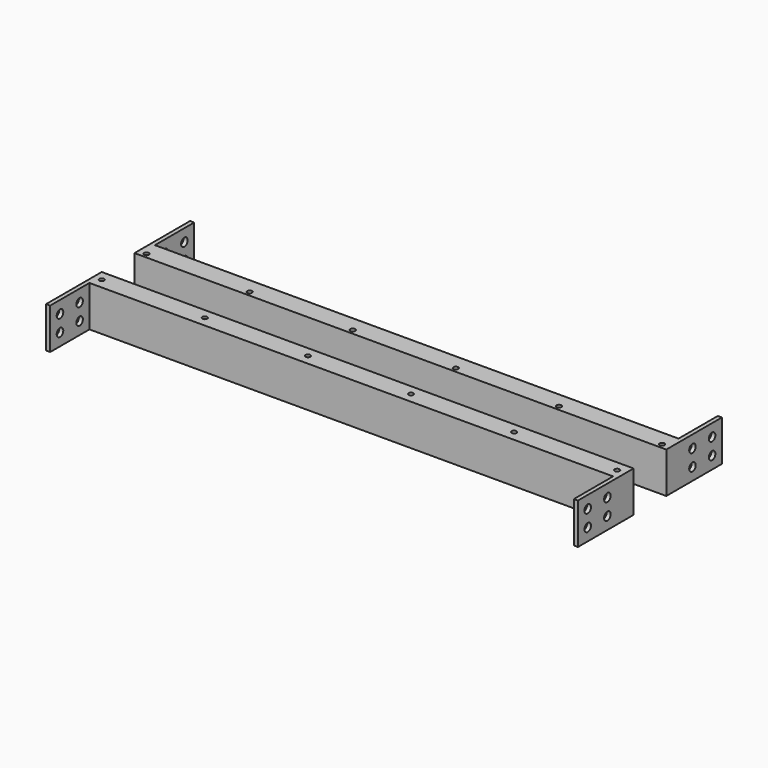
from build123d import *

# Parameters (mm, degrees)
F0_W      = 640
F0_H      = 50
F1_DEPTH  = 25
F2_W      = 19
F2_H      = 44
F3_DEPTH  = 1130
F4_W      = 85
F4_H      = 50
F5_DEPTH  = 5
F6_R      = 5
F7_DEPTH  = 5
F10_R     = 3
F11_DEPTH = 50
F12_R     = 3
F13_DEPTH = 50


# Not quite as in the source:
# - a pattern or mirror of a feature is missing from the dataset's text; its kind, count and spacing are read off the source's solid


with BuildPart() as f1:
    # F0 (on Front) → F1 (new body)
    with BuildSketch(Plane.XZ):
        Rectangle(F0_W, F0_H)
    extrude(amount=F1_DEPTH)

    # F2 (on face) → F3 (cut)
    with BuildSketch(Plane(origin=(-320, 0, 0), x_dir=(0, -1, 0), z_dir=(-1, 0, 0))):
        with Locations((12.5, 0)):
            Rectangle(F2_W, F2_H)
    extrude(amount=-F3_DEPTH, mode=Mode.SUBTRACT)

    # F4 (on face) → F5 (join)
    with BuildSketch(Plane(origin=(-320, 0, 0), x_dir=(0, -1, 0), z_dir=(-1, 0, 0))):
        with Locations((42.5, 0)):
            Rectangle(F4_W, F4_H)
    f5 = extrude(amount=F5_DEPTH)

    # F5_copies: F5 across plane
    add(f5.mirror(Plane(origin=(0, 0, 0), x_dir=(0, 0, 1), z_dir=(1, 0, 0))))

    # F6 (on face) → F7 (cut)
    with BuildSketch(Plane(origin=(-325, 0, 0), x_dir=(0, -1, 0), z_dir=(-1, 0, 0))):
        with Locations((40, -10)):
            Circle(F6_R)
        with Locations((40, 10)):
            Circle(F6_R)
        with Locations((70, 10)):
            Circle(F6_R)
        with Locations((70, -10)):
            Circle(F6_R)
    f7 = extrude(amount=-F7_DEPTH, mode=Mode.SUBTRACT)

    # F7_copies: F7 across plane
    add(f7.mirror(Plane(origin=(0, 0, 0), x_dir=(0, 0, 1), z_dir=(1, 0, 0))), mode=Mode.SUBTRACT)


with BuildPart() as f9_1:
    # F9: instance of F1
    add(f1.part.mirror(Plane.XZ.offset(-25)))

    # F12 (on face) → F13 (cut)
    with BuildSketch(Plane.XY.offset(25)):
        with Locations((-315, 56)):
            Circle(F12_R)
        with Locations((-189, 56)):
            Circle(F12_R)
        with Locations((-63, 56)):
            Circle(F12_R)
        with Locations((63, 56)):
            Circle(F12_R)
        with Locations((189, 56)):
            Circle(F12_R)
        with Locations((315, 56)):
            Circle(F12_R)
    extrude(amount=-F13_DEPTH, mode=Mode.SUBTRACT)


with BuildPart() as f1_1:
    add(f1.part)

    # F10 (on face) → F11 (cut)
    with BuildSketch(Plane.XY.offset(25)):
        with Locations((-315, -12.5)):
            Circle(F10_R)
        with Locations((-189, -12.5)):
            Circle(F10_R)
        with Locations((-63, -12.5)):
            Circle(F10_R)
        with Locations((63, -12.5)):
            Circle(F10_R)
        with Locations((189, -12.5)):
            Circle(F10_R)
        with Locations((315, -12.5)):
            Circle(F10_R)
    extrude(amount=-F11_DEPTH, mode=Mode.SUBTRACT)


solid = Compound([f9_1.part, f1_1.part])
